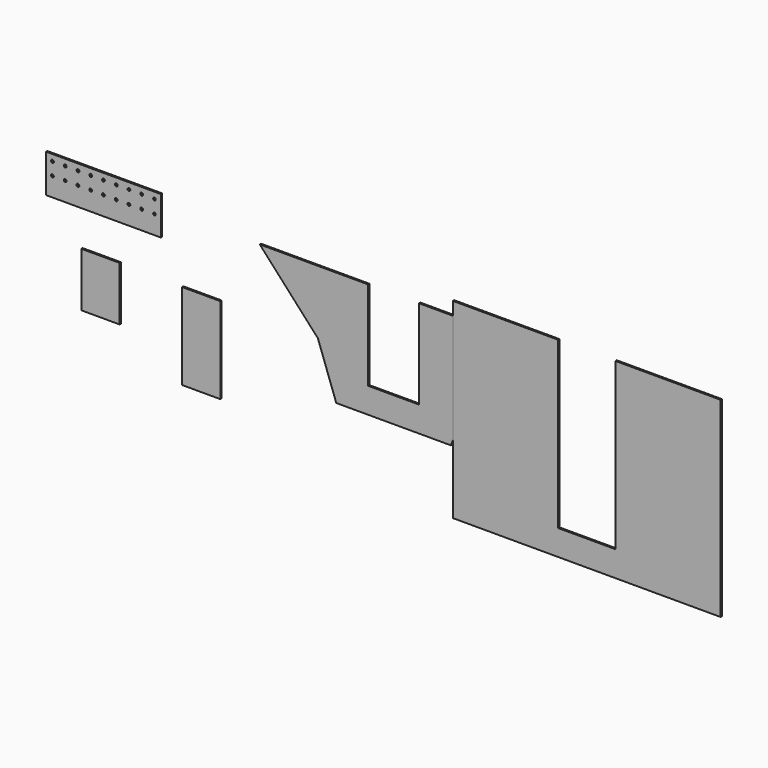
from build123d import *

# Parameters (mm, degrees)
F1_DEPTH = 3.175
F4_W     = 76.2
F4_H     = 107.96778
F6_DEPTH = 3.175
F5_W     = 76.2
F5_H     = 171.91228
F7_DEPTH = 3.175
F3_W     = 228.6
F3_H     = 76.2
F3_R     = 2.794
F3_R_2   = 2.54
F8_DEPTH = 3.175
F9_DEPTH = 3.175


# Not quite as in the source:
# - a length typed as a fraction of an inch, garbled in the dataset ("3 / 203.2 mm" for 3/8 in), is restored


with BuildPart() as f1:
    # F0 (on Front) → F1 (new body)
    with BuildSketch(Plane.XZ):
        Polygon((-217.3804237127, 143.8863651395), (-433.2804237127, 143.8863651395), (-317.4146833124, 16.8863651395), (-280.8804237127, -84.7136348605), (-52.2804237127, -84.7136348605), (-15.7461641131, 16.8863651395), (100.1195762873, 143.8863651395), (-115.7804237127, 143.8863651395), (-115.7804237127, -33.9136348605), (-217.3804237127, -33.9136348605), align=None)
    extrude(amount=F1_DEPTH)


with BuildPart() as f6:
    # F4 (on Front) → F6 (new body)
    with BuildSketch(Plane.XZ):
        with Locations((-750.7039308548, -33.3585813642)):
            Rectangle(F4_W, F4_H)
    extrude(amount=F6_DEPTH)


with BuildPart() as f7:
    # F5 (on Front) → F7 (new body)
    with BuildSketch(Plane.XZ):
        with Locations((-550.0105619431, -67.1462193131)):
            Rectangle(F5_W, F5_H)
    extrude(amount=F7_DEPTH)


with BuildPart() as f8:
    # F3 (on Front) → F8 (new body)
    with BuildSketch(Plane.XZ):
        with Locations((-744.705254101, 129.9696020692)):
            Rectangle(F3_W, F3_H)
        with Locations((-846.3592469164, 129.9158378293)):
            Circle(F3_R, mode=Mode.SUBTRACT)
        with Locations((-820.9594754919, 129.808080774)):
            Circle(F3_R, mode=Mode.SUBTRACT)
        with Locations((-795.5597040674, 129.7003237186)):
            Circle(F3_R, mode=Mode.SUBTRACT)
        with Locations((-770.1599326429, 129.5925666632)):
            Circle(F3_R, mode=Mode.SUBTRACT)
        with Locations((-744.7601612184, 129.4848096079)):
            Circle(F3_R, mode=Mode.SUBTRACT)
        with Locations((-719.3603897939, 129.3770525525)):
            Circle(F3_R, mode=Mode.SUBTRACT)
        with Locations((-693.9606183694, 129.2692954972)):
            Circle(F3_R, mode=Mode.SUBTRACT)
        with Locations((-668.5608469449, 129.1615384418)):
            Circle(F3_R, mode=Mode.SUBTRACT)
        with Locations((-643.1610755204, 129.0537813865)):
            Circle(F3_R_2, mode=Mode.SUBTRACT)
        with Locations((-846.305254101, 155.3696020692)):
            Circle(F3_R, mode=Mode.SUBTRACT)
        with Locations((-820.905254101, 155.3696020692)):
            Circle(F3_R, mode=Mode.SUBTRACT)
        with Locations((-795.505254101, 155.3696020692)):
            Circle(F3_R, mode=Mode.SUBTRACT)
        with Locations((-770.105254101, 155.3696020692)):
            Circle(F3_R, mode=Mode.SUBTRACT)
        with Locations((-744.705254101, 155.3696020692)):
            Circle(F3_R, mode=Mode.SUBTRACT)
        with Locations((-719.305254101, 155.3696020692)):
            Circle(F3_R, mode=Mode.SUBTRACT)
        with Locations((-693.905254101, 155.3696020692)):
            Circle(F3_R, mode=Mode.SUBTRACT)
        with Locations((-668.505254101, 155.3696020692)):
            Circle(F3_R, mode=Mode.SUBTRACT)
        with Locations((-643.105254101, 155.3696020692)):
            Circle(F3_R_2, mode=Mode.SUBTRACT)
    extrude(amount=F8_DEPTH)


with BuildPart() as f9:
    # F2 (on Front) → F9 (new body)
    with BuildSketch(Plane.XZ):
        Polygon((161.1693713427, 169.9292318031), (-48.3806286573, 169.9292318031), (-48.3806286573, -211.0707681969), (485.0193713427, -211.0707681969), (485.0193713427, 169.9292318031), (275.4693713427, 169.9292318031), (275.4693713427, -160.2707681969), (161.1693713427, -160.2707681969), align=None)
    extrude(amount=F9_DEPTH)


solid = Compound([f1.part, f6.part, f7.part, f8.part, f9.part])
